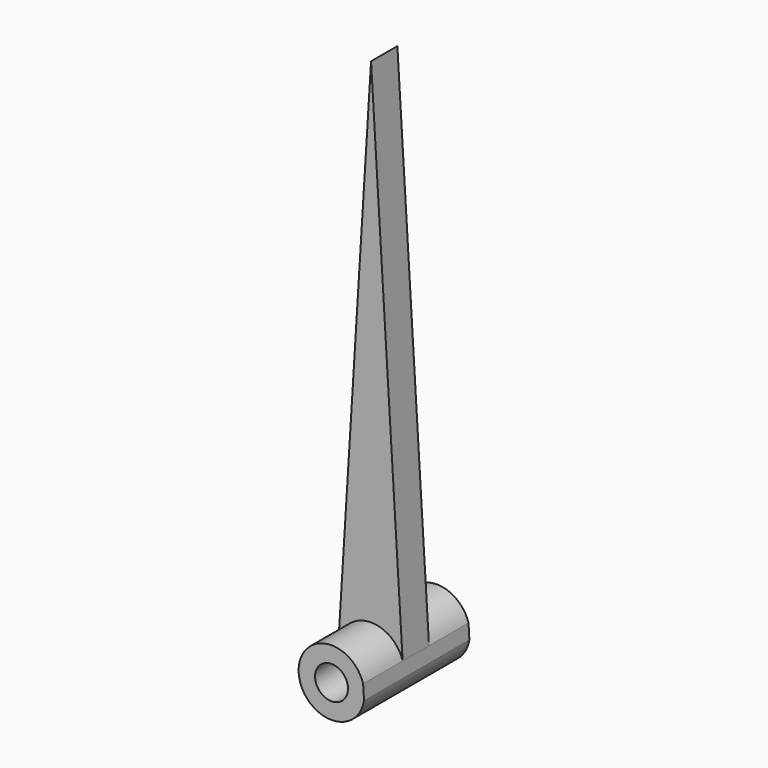
from build123d import *

# Parameters (mm, degrees)
F0_R     = 1.5875
F1_DEPTH = 6.35
F2_DEPTH = 1.5875


with BuildPart() as f1:
    # F0 (on Front) → F1 (new body, symmetric)
    with BuildSketch(Plane.XZ):
        with BuildLine():
            ThreePointArc((-3.1749141346, 0.0233503235), (-0.2706319367, -3.1634448557), (3.1327451143, -0.5162683885))
            Line((3.1327451143, -0.5162683885), (3.0466813259, 0.8935087569))
            ThreePointArc((3.0466813259, 0.8935087569), (-0.2659699045, 3.1638402314), (-3.153094005, 0.3723213606))
            Line((-3.153094005, 0.3723213606), (-3.1749141346, 0.0233503235))
        make_face()
        Circle(F0_R, mode=Mode.SUBTRACT)
    extrude(amount=F1_DEPTH, both=True)

    # F0 (on Front) → F2 (join, symmetric)
    with BuildSketch(Plane.XZ):
        with BuildLine():
            ThreePointArc((-3.153094005, 0.3723213606), (-0.2659699045, 3.1638402314), (3.0466813259, 0.8935087569))
            Line((3.0466813259, 0.8935087569), (0, 50.8))
            Line((0, 50.8), (-3.153094005, 0.3723213606))
        make_face()
    extrude(amount=F2_DEPTH, both=True)


solid = f1.part
